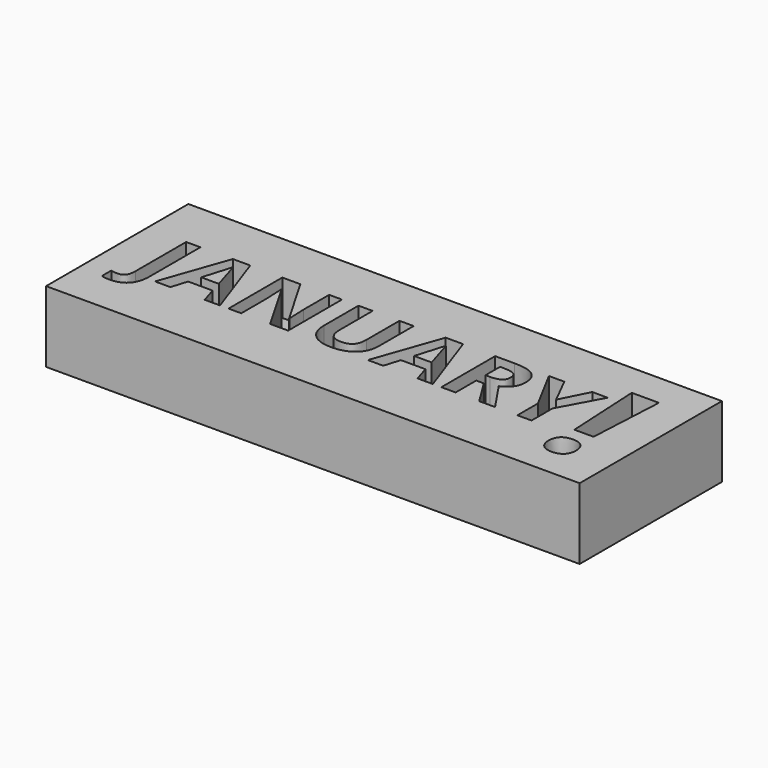
from build123d import *

# Parameters (mm, degrees)
F0_W         = 38.1
F0_H         = 12.7
F1_DEPTH     = 5.08
F2_TEXT_SIZE = 6.7275664252
F3_DEPTH     = 2.54
F4_TEXT_SIZE = 11.4861979253
F5_DEPTH     = 2.54


# Not quite as in the source:
# - Text() gives the source's letters only with a copy of the font that has no kerning and outlines rounded to 1/6400 em; it was checked with that copy


with BuildPart() as f1:
    # F0 (on Top) → F1 (new body)
    with BuildSketch(Plane.XY):
        with Locations((34.9995701134, -27.7311721981)):
            Rectangle(F0_W, F0_H)
    extrude(amount=F1_DEPTH)

    # F2 (on face) → F3 (cut)
    with BuildSketch(Plane.XY.offset(5.08)):
        with Locations((18.1135758758, -29.8452991992)):
            Text('JANUARY', F2_TEXT_SIZE, font='Open Sans', font_style=FontStyle.BOLD, text_align=(TextAlign.LEFT, TextAlign.BOTTOM))
    extrude(amount=-F3_DEPTH, mode=Mode.SUBTRACT)

    # F4 (on face) → F5 (cut)
    with BuildSketch(Plane.XY.offset(5.08)):
        with Locations((48.8196606954, -31.9397076964)):
            Text('!', F4_TEXT_SIZE, font='Open Sans', font_style=FontStyle.BOLD, text_align=(TextAlign.LEFT, TextAlign.BOTTOM))
    extrude(amount=-F5_DEPTH, mode=Mode.SUBTRACT)


solid = f1.part
